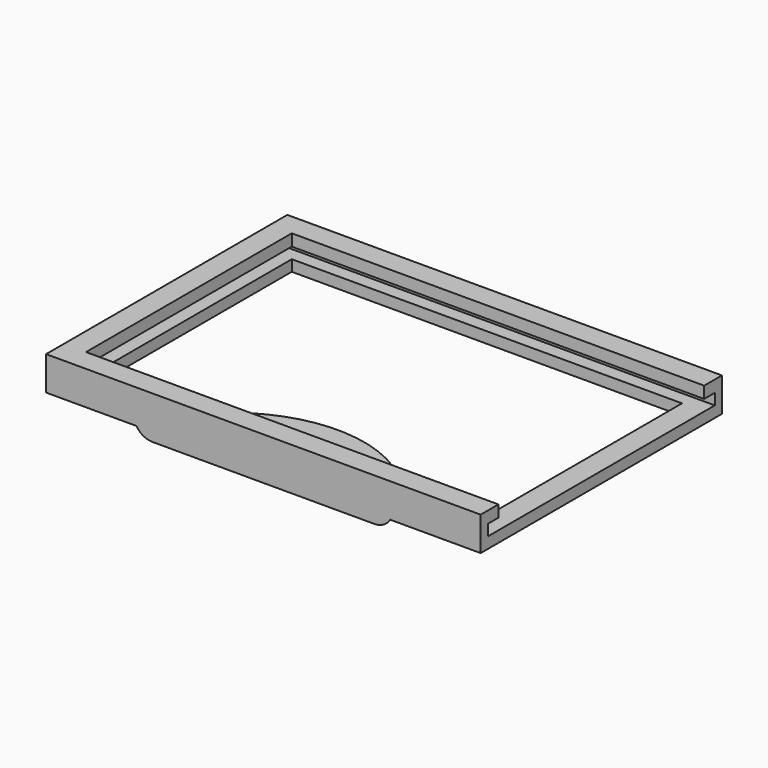
from build123d import *

# Parameters (mm, degrees)
F0_W        = 2.54
F0_H        = 3.81
F0_W_2      = 3.81
F0_H_2      = 73.66
F1_DEPTH    = 3.175
F2_DEPTH    = 9.7028
F3_START    = 6.35
F3_DEPTH    = 3.3528
F5_DEPTH    = 2.54
F6_T2_ANGLE = 26.9228721227
F6_T4_ANGLE = 124.2205290786
F6_T6_ANGLE = 26.9228721227


# Not quite as in the source:
# - a fillet or chamfer that OpenCascade refuses, or shapes differently, is made with other operations: its cross-section is extruded or revolved along the edge and cut away or added


with BuildPart() as f1:
    # F0 (on Top) → F1 (new body)
    with BuildSketch(Plane.XY):
        Polygon((-55.88, -36.83), (-55.88, 36.83), (55.88, 36.83), (59.69, 36.83), (59.69, 40.64), (-59.69, 40.64), (-59.69, -40.64), (59.69, -40.64), (59.69, -36.83), (55.88, -36.83), align=None)
        with Locations((60.96, 38.735)):
            Rectangle(F0_W, F0_H)
        with Locations((60.96, -38.735)):
            Rectangle(F0_W, F0_H)
        with Locations((57.785, 0)):
            Rectangle(F0_W_2, F0_H_2)
        with Locations((60.96, 0)):
            Rectangle(F0_W, F0_H_2)
    extrude(amount=F1_DEPTH)

    # F0 (on Top) → F2 (join)
    with BuildSketch(Plane.XY):
        Polygon((-59.69, 40.64), (59.69, 40.64), (62.23, 40.64), (62.23, 43.18), (-62.23, 43.18), (-62.23, -43.18), (62.23, -43.18), (62.23, -40.64), (59.69, -40.64), (-59.69, -40.64), align=None)
    extrude(amount=F2_DEPTH)

    # F0 (on Top) → F3 (join)
    with BuildSketch(Plane.XY.offset(F3_START)):
        Polygon((-55.88, -36.83), (-55.88, 36.83), (55.88, 36.83), (59.69, 36.83), (59.69, 40.64), (-59.69, 40.64), (-59.69, -40.64), (59.69, -40.64), (59.69, -36.83), (55.88, -36.83), align=None)
        with Locations((60.96, -38.735)):
            Rectangle(F0_W, F0_H)
        with Locations((60.96, 38.735)):
            Rectangle(F0_W, F0_H)
    extrude(amount=F3_DEPTH)

    # F4 (on face) → F5 (join)
    with BuildSketch(Plane(origin=(0, 0, 0), x_dir=(1, 0, 0), z_dir=(0, 0, -1))):
        with BuildLine():
            Line((33.6746639179, 36.83), (-33.6746639179, 36.83))
            ThreePointArc((-33.6746639179, 36.83), (0, 16.5520933119), (33.6746639179, 36.83))
        make_face()
        with BuildLine():
            Line((36.331819044, 43.18), (-36.331819044, 43.18))
            ThreePointArc((-36.331819044, 43.18), (-35.1469421027, 39.9448685285), (-33.6746639179, 36.83))
            Line((-33.6746639179, 36.83), (33.6746639179, 36.83))
            ThreePointArc((33.6746639179, 36.83), (35.1469421027, 39.9448685285), (36.331819044, 43.18))
        make_face()
    extrude(amount=F5_DEPTH)

    # F6: fillet of radius 5.08 on 1 edges, made by hand

    # F6_s1 → F6_t2 (revolve, cut)
    with BuildSketch(Plane(origin=(-0.9220761964, -54.6365318462, 0), x_dir=(0, 0, 1), z_dir=(-0.0168741478, -0.9998576214, 0))):
        with BuildLine():
            ThreePointArc((0, 37.177792501), (-1.8594090512, 35.3183834498), (-2.54, 32.7783834498))
            Line((-2.54, 32.7783834498), (-2.54, 37.177792501))
            Line((-2.54, 37.177792501), (0, 37.177792501))
        make_face()
    revolve(axis=Axis((0, -54.6520933119, -2.54), (0, 0, -1)), revolution_arc=F6_T2_ANGLE, mode=Mode.SUBTRACT)

    # F6_s3 → F6_t4 (revolve, cut)
    with BuildSketch(Plane(origin=(-22.5953375952, -42.6936601597, 0), x_dir=(0, 0, 1), z_dir=(-0.4677714801, -0.8838494455, 0))):
        with BuildLine():
            ThreePointArc((0, 12.5353094191), (-1.8594090512, 10.6759003679), (-2.54, 8.1359003679))
            Line((-2.54, 8.1359003679), (-2.54, 12.5353094191))
            Line((-2.54, 12.5353094191), (0, 12.5353094191))
        make_face()
    revolve(axis=Axis((0, -54.6520933119, -2.54), (0, 0, -1)), revolution_arc=F6_T4_ANGLE, mode=Mode.SUBTRACT)

    # F6_s5 → F6_t6 (revolve, cut)
    with BuildSketch(Plane(origin=(22.5953375952, -42.6936601597, 0), x_dir=(0, 0, 1), z_dir=(-0.4677714801, 0.8838494455, 0))):
        with BuildLine():
            ThreePointArc((0, 12.5353094191), (-1.8594090512, 10.6759003679), (-2.54, 8.1359003679))
            Line((-2.54, 8.1359003679), (-2.54, 12.5353094191))
            Line((-2.54, 12.5353094191), (0, 12.5353094191))
        make_face()
    revolve(axis=Axis((0, -54.6520933119, -2.54), (0, 0, -1)), revolution_arc=F6_T6_ANGLE, mode=Mode.SUBTRACT)


solid = f1.part
